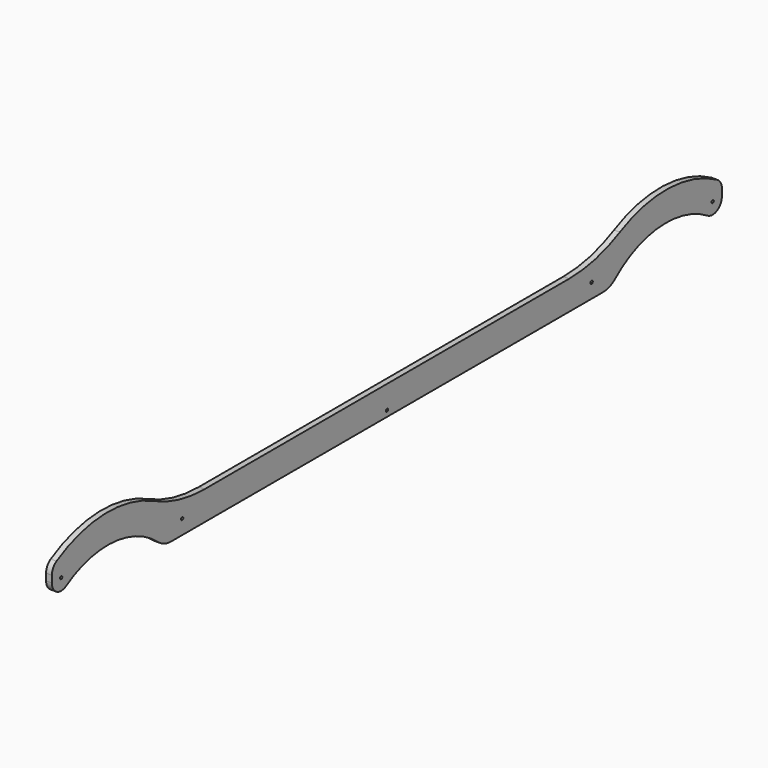
from build123d import *

# Parameters (mm, degrees)
F1_DEPTH      = 12.7
F2_R          = 3.175
F3_DEPTH      = 25.4
F3_DEPTH_BACK = 1882


# Not quite as in the source:
# - an extrude ends at something that could not be found from the text; its depth is read off the source's solid


with BuildPart() as f1:
    # F0 (on Right) → F1 (new body)
    with BuildSketch(Plane.YZ):
        with BuildLine():
            ThreePointArc((-622.6993794949, 12.1531100478), (-607.2983658108, 3.1350127999), (-589.7288184286, 0))
            Line((-589.7288184286, 0), (589.7288184286, 0))
            ThreePointArc((589.7288184286, 0), (607.2983658108, 3.1350127999), (622.6993794949, 12.1531100478))
            ThreePointArc((622.6993794949, 12.1531100478), (746.0500791914, 62.9065317561), (875.5608465608, 30.9962502452))
            ThreePointArc((875.5608465608, 30.9962502452), (901.3248834202, 30.3402571366), (914.4, 52.5496526411))
            Line((914.4, 52.5496526411), (914.4, 67.3727526142))
            ThreePointArc((914.4, 67.3727526142), (911.0154605337, 80.0408028781), (901.7638190955, 89.3328282539))
            ThreePointArc((901.7638190955, 89.3328282539), (769.7029358002, 126.8933113968), (635.7649329622, 96.7026143791))
            ThreePointArc((635.7649329622, 96.7026143791), (568.5593617374, 71.9168669296), (497.4251334688, 63.5))
            Line((497.4251334688, 63.5), (-497.4251334688, 63.5))
            ThreePointArc((-497.4251334688, 63.5), (-568.5593617374, 71.9168669296), (-635.7649329622, 96.7026143791))
            ThreePointArc((-635.7649329622, 96.7026143791), (-769.7029358002, 126.8933113968), (-901.7638190955, 89.3328282539))
            ThreePointArc((-901.7638190955, 89.3328282539), (-911.0154605337, 80.0408028781), (-914.4, 67.3727526142))
            Line((-914.4, 67.3727526142), (-914.4, 52.5496526411))
            ThreePointArc((-914.4, 52.5496526411), (-901.3248834202, 30.3402571366), (-875.5608465608, 30.9962502452))
            ThreePointArc((-875.5608465608, 30.9962502452), (-746.0500791914, 62.9065317561), (-622.6993794949, 12.1531100478))
        make_face()
    extrude(amount=F1_DEPTH)

    # F2 (on face) → F3 (cut, two sides)
    with BuildSketch(Plane.YZ.offset(12.7)) as f3_sk:
        with Locations((-889, 52.5496526411)):
            Circle(F2_R)
        with Locations((-558.8, 31.75)):
            Circle(F2_R)
        with Locations((0, 12.7)):
            Circle(F2_R)
        with Locations((558.8, 31.75)):
            Circle(F2_R)
        with Locations((889, 52.5496526411)):
            Circle(F2_R)
    extrude(amount=-F3_DEPTH, mode=Mode.SUBTRACT)
    extrude(f3_sk.sketch, amount=F3_DEPTH_BACK, mode=Mode.SUBTRACT)


solid = f1.part
